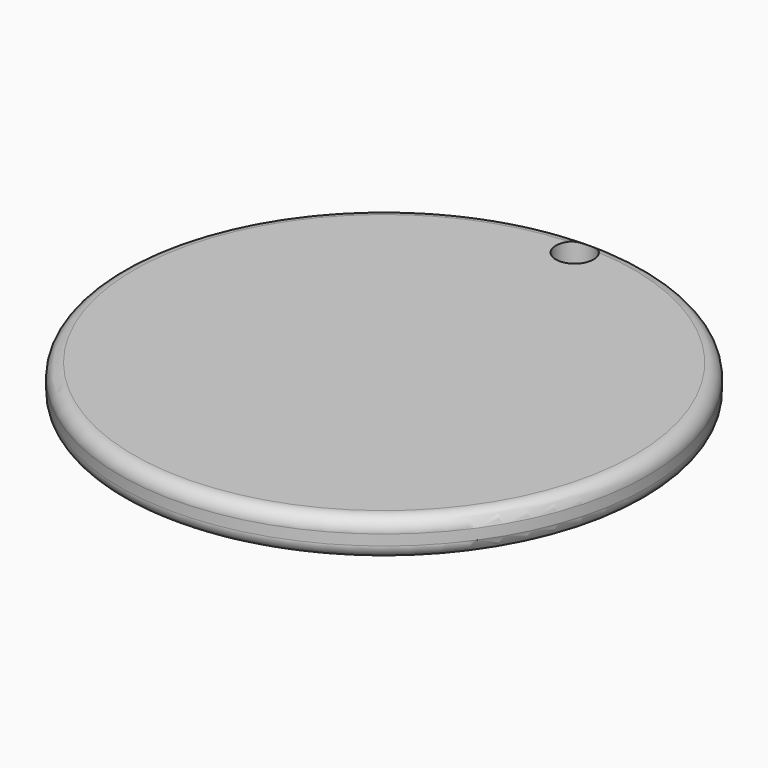
from build123d import *

# Parameters (mm, degrees)
F0_R     = 44.45
F1_DEPTH = 3.175
F2_R     = 3.175
F3_DEPTH = 12.7


# Not quite as in the source:
# - a fillet or chamfer that OpenCascade refuses, or shapes differently, is made with other operations: its cross-section is extruded or revolved along the edge and cut away or added


with BuildPart() as f1:
    # F0 (on Top) → F1 (new body, symmetric)
    with BuildSketch(Plane.XY):
        Circle(F0_R)
    extrude(amount=F1_DEPTH, both=True)

    # F2 (on Top) → F3 (cut, symmetric)
    with BuildSketch(Plane.XY):
        with Locations((0, 40.1277458341)):
            Circle(F2_R)
    extrude(amount=F3_DEPTH, both=True, mode=Mode.SUBTRACT)

    # F4: fillet of radius 2.286 on 2 edges, made by hand

    # F4_s1 → F4_t2 (revolve, cut)
    with BuildSketch(Plane.XZ):
        with BuildLine():
            ThreePointArc((44.45, 0.889), (43.7804461018, 2.5054461018), (42.164, 3.175))
            Line((42.164, 3.175), (44.45, 3.175))
            Line((44.45, 3.175), (44.45, 0.889))
        make_face()
    revolve(axis=Axis((0, 0, 3.175), (0, 0, 1)), mode=Mode.SUBTRACT)

    # F4_s3 → F4_t4 (revolve, cut)
    with BuildSketch(Plane.XZ):
        with BuildLine():
            ThreePointArc((44.45, -0.889), (43.7804461018, -2.5054461018), (42.164, -3.175))
            Line((42.164, -3.175), (44.45, -3.175))
            Line((44.45, -3.175), (44.45, -0.889))
        make_face()
    revolve(axis=Axis((0, 0, -3.175), (0, 0, 1)), mode=Mode.SUBTRACT)


solid = f1.part
